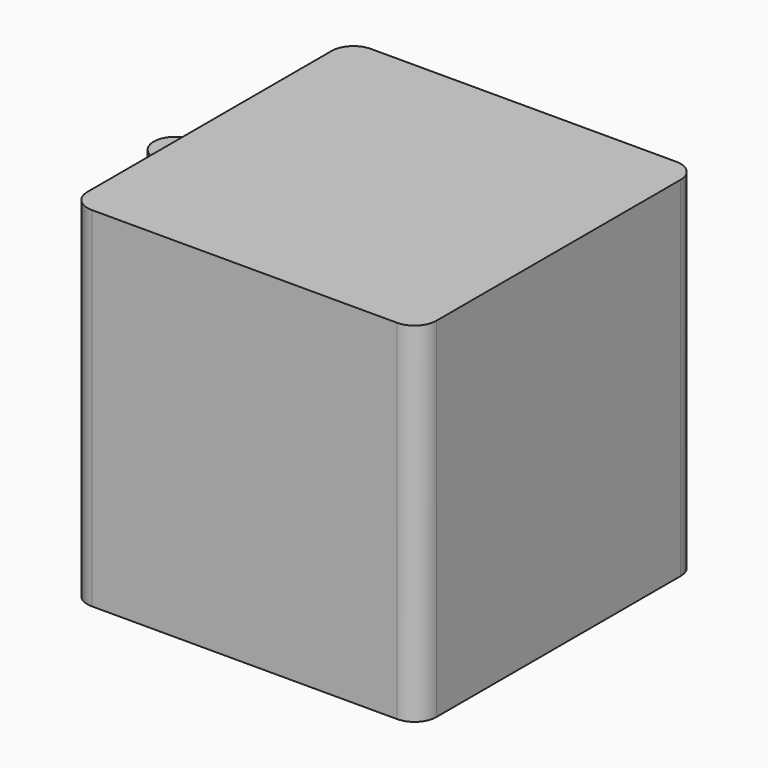
from build123d import *

# Parameters (mm, degrees)
F0_W      = 25.4
F0_H      = 25.4
F1_DEPTH  = 3.175
F2_W      = 25.4
F2_H      = 25.4
F3_DEPTH  = 1.5875
F4_R      = 10
F5_DEPTH  = 1
F6_R      = 9
F7_DEPTH  = 88
F8_R      = 10
F8_R_2    = 9
F9_DEPTH  = 88
F10_R     = 10
F11_DEPTH = 1
F12_W     = 160
F12_H     = 160
F13_DEPTH = 160
F14_R     = 10


with BuildPart() as f1:
    # F0 (on Top) → F1 (new body)
    with BuildSketch(Plane.XY):
        Rectangle(F0_W, F0_H)
    extrude(amount=F1_DEPTH)


with BuildPart() as f3:
    # F2 (on face) → F3 (new body)
    with BuildSketch(Plane.XY.offset(3.175)):
        Rectangle(F2_W, F2_H)
    extrude(amount=F3_DEPTH)


with BuildPart() as f5:
    # F4 (on Top) → F5 (new body)
    with BuildSketch(Plane.XY):
        with Locations((-47.0507442951, -28.9763715118)):
            Circle(F4_R)
    extrude(amount=F5_DEPTH)

    # F6 (on face) → F7 (join)
    with BuildSketch(Plane.XY.offset(1)):
        with Locations((-47.0507442951, -28.9763715118)):
            Circle(F6_R)
    extrude(amount=F7_DEPTH)


with BuildPart() as f9:
    # F8 (on face) → F9 (new body, through all)
    with BuildSketch(Plane.XY.offset(1)):
        with Locations((-47.0507442951, -28.9763715118)):
            Circle(F8_R)
        with Locations((-47.0507442951, -28.9763715118)):
            Circle(F8_R_2, mode=Mode.SUBTRACT)
    extrude(amount=F9_DEPTH)

    # F10 (on face) → F11 (join)
    with BuildSketch(Plane.XY.offset(89)):
        with Locations((-47.0507442951, -28.9763715118)):
            Circle(F10_R)
    extrude(amount=F11_DEPTH)


with BuildPart() as f13:
    # F12 (on Top) → F13 (new body)
    with BuildSketch(Plane.XY):
        with Locations((112.7631608397, -109.2488616705)):
            Rectangle(F12_W, F12_H)
    extrude(amount=F13_DEPTH)

    # F14
    f14_edges = [f13.edges().sort_by_distance(p)[0] for p in [
        (32.763161, -189.248862, 80),
        (192.763161, -189.248862, 80),
        (192.763161, -29.248862, 80),
        (32.763161, -29.248862, 80),
    ]]
    fillet(f14_edges, radius=F14_R)


solid = Compound([f1.part, f3.part, f5.part, f9.part, f13.part])
